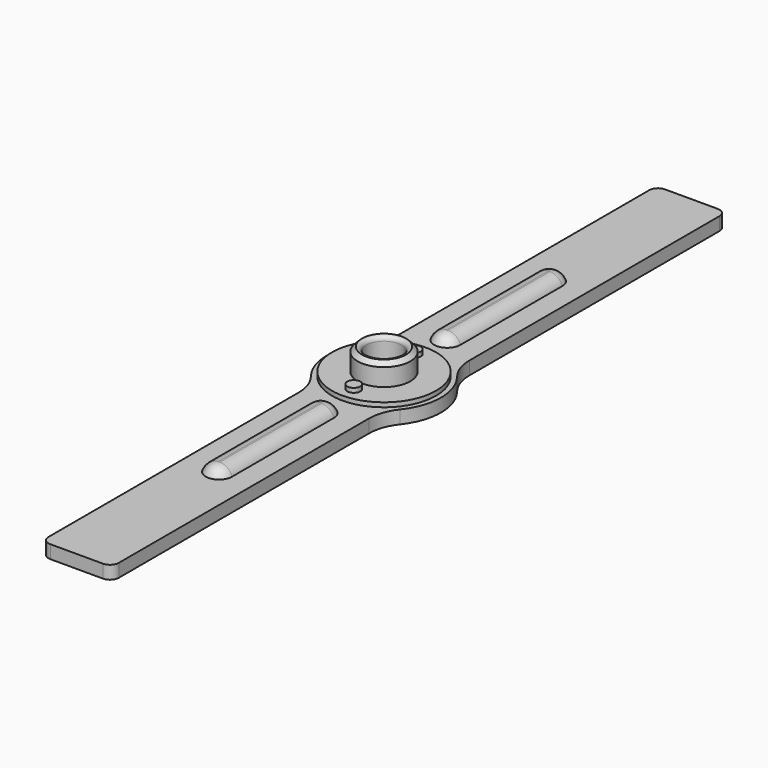
from build123d import *

# Parameters (mm, degrees)
F1_DEPTH      = 0.762
F2_R          = 2.54
F3_R          = 0.508
F4_R          = 3.0139316414
F5_DEPTH      = 0.254
F6_R          = 1.524
F7_DEPTH      = 1.27
F8_SIZE       = 0.254
F9_R          = 0.381
F10_DEPTH     = 0.254
F11_R         = 1.016
F12_DEPTH     = 25.4
F13_R         = 0.25399
F15_DEPTH     = 0.508
F16_T1_DEPTH  = 7.366
F16_T3_DEPTH  = 7.366
F16_T6_ANGLE  = 180
F16_T8_ANGLE  = 180
F16_T10_ANGLE = 180
F16_T12_ANGLE = 180


# Not quite as in the source:
# - a fillet or chamfer that OpenCascade refuses, or shapes differently, is made with other operations: its cross-section is extruded or revolved along the edge and cut away or added
# - a fillet or chamfer is up to 0.001 mm smaller than in the source, because OpenCascade refuses the exact size


with BuildPart() as f1:
    # F0 (on Top) → F1 (new body)
    with BuildSketch(Plane.XY):
        with BuildLine():
            Line((2.032, -14.605), (2.032, -2.6027254946))
            ThreePointArc((2.032, -2.6027254946), (3.302, 0), (2.032, 2.6027254946))
            Line((2.032, 2.6027254946), (2.032, 14.605))
            Line((2.032, 14.605), (2.032, 22.225))
            Line((2.032, 22.225), (-2.032, 22.225))
            Line((-2.032, 22.225), (-2.032, 14.605))
            Line((-2.032, 14.605), (-2.032, 2.6027254946))
            ThreePointArc((-2.032, 2.6027254946), (-3.302, 0), (-2.032, -2.6027254946))
            Line((-2.032, -2.6027254946), (-2.032, -14.605))
            Line((-2.032, -14.605), (-2.032, -22.225))
            Line((-2.032, -22.225), (2.032, -22.225))
            Line((2.032, -22.225), (2.032, -14.605))
        make_face()
    extrude(amount=F1_DEPTH)

    # F2
    f2_edges = [f1.edges().sort_by_distance(p)[0] for p in [
        (-2.032, 2.602725, 0.381),
        (-2.032, -2.602725, 0.381),
        (2.032, 2.602725, 0.381),
        (2.032, -2.602725, 0.381),
    ]]
    fillet(f2_edges, radius=F2_R)

    # F3
    f3_edges = [f1.edges().sort_by_distance(p)[0] for p in [
        (-2.032, -22.225, 0.381),
        (2.032, -22.225, 0.381),
        (-2.032, 22.225, 0.381),
        (2.032, 22.225, 0.381),
    ]]
    fillet(f3_edges, radius=F3_R)

    # F4 (on face) → F5 (join)
    with BuildSketch(Plane.XY.offset(0.762)):
        Circle(F4_R)
    extrude(amount=F5_DEPTH)

    # F6 (on face) → F7 (join)
    with BuildSketch(Plane.XY.offset(1.016)):
        Circle(F6_R)
    extrude(amount=F7_DEPTH)

    # F8
    f8_edges = [f1.edges().sort_by_distance(p)[0] for p in [
        (-1.524, 0, 2.286),
    ]]
    chamfer(f8_edges, length=F8_SIZE)

    # F9 (on face) → F10 (join)
    with BuildSketch(Plane.XY.offset(1.016)):
        with Locations((0, 2.1844)):
            Circle(F9_R)
        with Locations((0, -2.1844)):
            Circle(F9_R)
    extrude(amount=F10_DEPTH)

    # F11 (on face) → F12 (cut)
    with BuildSketch(Plane.XY.offset(2.286)):
        Circle(F11_R)
    extrude(amount=-F12_DEPTH, mode=Mode.SUBTRACT)

    # F13 (radius 0.254 in the source; OpenCascade refuses exactly that, so slightly less here)
    f13_edges = [f1.edges().sort_by_distance(p)[0] for p in [
        (-1.016, 0, 2.286),
        (-1.016, 0, 0),
    ]]
    fillet(f13_edges, radius=F13_R)

    # F14 (on face) → F15 (join)
    with BuildSketch(Plane.XY.offset(0.762)):
        with BuildLine():
            ThreePointArc((0, 12.7), (-0.5388153673, 12.4768153673), (-0.762, 11.938))
            Line((-0.762, 11.938), (-0.762, 4.572))
            ThreePointArc((-0.762, 4.572), (-0.5388153673, 4.0331846327), (0, 3.81))
            ThreePointArc((0, 3.81), (0.5388153673, 4.0331846327), (0.762, 4.572))
            Line((0.762, 4.572), (0.762, 11.938))
            ThreePointArc((0.762, 11.938), (0.5388153673, 12.4768153673), (0, 12.7))
        make_face()
        with BuildLine():
            ThreePointArc((0, -3.81), (-0.5388153673, -4.0331846327), (-0.762, -4.572))
            Line((-0.762, -4.572), (-0.762, -11.938))
            ThreePointArc((-0.762, -11.938), (-0.5388153673, -12.4768153673), (0, -12.7))
            ThreePointArc((0, -12.7), (0.5388153673, -12.4768153673), (0.762, -11.938))
            Line((0.762, -11.938), (0.762, -4.572))
            ThreePointArc((0.762, -4.572), (0.5388153673, -4.0331846327), (0, -3.81))
        make_face()
    extrude(amount=F15_DEPTH)

    # F16: fillet of radius 0.762 on 8 edges, made by hand

    # F16_s2 → F16_t1 (cut)
    with BuildSketch(Plane.XZ.offset(-11.938)):
        with BuildLine():
            ThreePointArc((-0.762, 0.762), (-0.4835204154, 1.1301703947), (-0.0435795103, 1.27))
            Line((-0.0435795103, 1.27), (-0.762, 1.27))
            Line((-0.762, 1.27), (-0.762, 0.762))
        make_face()
        with BuildLine():
            ThreePointArc((0.762, 0.762), (0.4835204154, 1.1301703947), (0.0435795103, 1.27))
            Line((0.0435795103, 1.27), (0.762, 1.27))
            Line((0.762, 1.27), (0.762, 0.762))
        make_face()
    extrude(amount=F16_T1_DEPTH, mode=Mode.SUBTRACT)

    # F16_s4 → F16_t3 (cut)
    with BuildSketch(Plane.XZ.offset(4.572)):
        with BuildLine():
            ThreePointArc((-0.762, 0.762), (-0.4835204154, 1.1301703947), (-0.0435795103, 1.27))
            Line((-0.0435795103, 1.27), (-0.762, 1.27))
            Line((-0.762, 1.27), (-0.762, 0.762))
        make_face()
        with BuildLine():
            ThreePointArc((0.762, 0.762), (0.4835204154, 1.1301703947), (0.0435795103, 1.27))
            Line((0.0435795103, 1.27), (0.762, 1.27))
            Line((0.762, 1.27), (0.762, 0.762))
        make_face()
    extrude(amount=F16_T3_DEPTH, mode=Mode.SUBTRACT)

    # F16_s5 → F16_t6 (revolve, cut)
    with BuildSketch(Plane.XZ.offset(-11.938)):
        with BuildLine():
            ThreePointArc((0.762, 0.762), (0.4835204154, 1.1301703947), (0.0435795103, 1.27))
            Line((0.0435795103, 1.27), (0.762, 1.27))
            Line((0.762, 1.27), (0.762, 0.762))
        make_face()
    revolve(axis=Axis((0, 11.938, 1.27), (0, 0, 1)), revolution_arc=F16_T6_ANGLE, mode=Mode.SUBTRACT)

    # F16_s7 → F16_t8 (revolve, cut)
    with BuildSketch(Plane.XZ.offset(-4.572)):
        with BuildLine():
            ThreePointArc((-0.762, 0.762), (-0.4835204154, 1.1301703947), (-0.0435795103, 1.27))
            Line((-0.0435795103, 1.27), (-0.762, 1.27))
            Line((-0.762, 1.27), (-0.762, 0.762))
        make_face()
    revolve(axis=Axis((0, 4.572, 1.27), (0, 0, 1)), revolution_arc=F16_T8_ANGLE, mode=Mode.SUBTRACT)

    # F16_s9 → F16_t10 (revolve, cut)
    with BuildSketch(Plane.XZ.offset(4.572)):
        with BuildLine():
            ThreePointArc((0.762, 0.762), (0.4835204154, 1.1301703947), (0.0435795103, 1.27))
            Line((0.0435795103, 1.27), (0.762, 1.27))
            Line((0.762, 1.27), (0.762, 0.762))
        make_face()
    revolve(axis=Axis((0, -4.572, 1.27), (0, 0, 1)), revolution_arc=F16_T10_ANGLE, mode=Mode.SUBTRACT)

    # F16_s11 → F16_t12 (revolve, cut)
    with BuildSketch(Plane.XZ.offset(11.938)):
        with BuildLine():
            ThreePointArc((-0.762, 0.762), (-0.4835204154, 1.1301703947), (-0.0435795103, 1.27))
            Line((-0.0435795103, 1.27), (-0.762, 1.27))
            Line((-0.762, 1.27), (-0.762, 0.762))
        make_face()
    revolve(axis=Axis((0, -11.938, 1.27), (0, 0, 1)), revolution_arc=F16_T12_ANGLE, mode=Mode.SUBTRACT)


solid = f1.part
